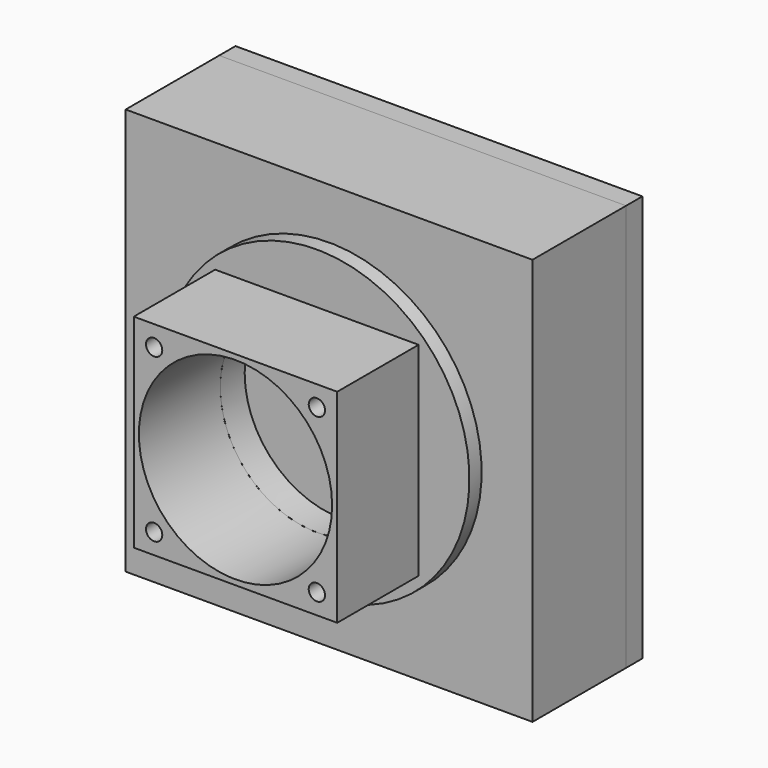
from build123d import *

# Parameters (mm, degrees)
F0_W      = 40
F0_H      = 40
F0_R      = 1.6
F0_R_2    = 19
F1_DEPTH  = 20
F2_R      = 30
F2_W      = 40
F2_H      = 40
F2_R_2    = 1.6
F2_R_3    = 19
F3_DEPTH  = 3
F4_W      = 80
F4_H      = 80
F4_R      = 30
F4_R_2    = 3
F4_R_3    = 19
F5_DEPTH  = 3
F6_W      = 80
F6_H      = 80
F6_W_2    = 76.0000017285
F6_H_2    = 76.0000017285
F7_DEPTH  = 20
F8_W      = 75.600002408
F8_H      = 75.600002408
F9_DEPTH  = 4
F8_W_2    = 80
F8_H_2    = 80
F8_W_3    = 76.0000017285
F8_H_3    = 76.0000017285
F10_DEPTH = 4


# Not quite as in the source:
# - a feature names something its author has since deleted; it is built from what else it names


with BuildPart() as f1:
    # F0 (on Front) → F1 (new body)
    with BuildSketch(Plane.XZ):
        Rectangle(F0_W, F0_H)
        with Locations((-16, -16)):
            Circle(F0_R, mode=Mode.SUBTRACT)
        with Locations((16, -16)):
            Circle(F0_R, mode=Mode.SUBTRACT)
        with Locations((-16, 16)):
            Circle(F0_R, mode=Mode.SUBTRACT)
        Circle(F0_R_2, mode=Mode.SUBTRACT)
        with Locations((16, 16)):
            Circle(F0_R, mode=Mode.SUBTRACT)
    extrude(amount=F1_DEPTH)


with BuildPart() as f3:
    # F2 (on face) → F3 (new body)
    with BuildSketch(Plane(origin=(0, 0, 0), x_dir=(-1, 0, 0), z_dir=(0, 1, 0))):
        Circle(F2_R)
        Rectangle(F2_W, F2_H, mode=Mode.SUBTRACT)
        Rectangle(F2_W, F2_H)
        with Locations((-16, -16)):
            Circle(F2_R_2, mode=Mode.SUBTRACT)
        with Locations((16, -16)):
            Circle(F2_R_2, mode=Mode.SUBTRACT)
        with Locations((-16, 16)):
            Circle(F2_R_2, mode=Mode.SUBTRACT)
        Circle(F2_R_3, mode=Mode.SUBTRACT)
        with Locations((16, 16)):
            Circle(F2_R_2, mode=Mode.SUBTRACT)
    extrude(amount=F3_DEPTH)

    # F4 (on face) → F5 (join)
    with BuildSketch(Plane(origin=(0, 3, 0), x_dir=(-1, 0, 0), z_dir=(0, 1, 0))):
        Rectangle(F4_W, F4_H)
        Circle(F4_R, mode=Mode.SUBTRACT)
        Circle(F4_R)
        with Locations((-16, -16)):
            Circle(F4_R_2, mode=Mode.SUBTRACT)
        with Locations((16, -16)):
            Circle(F4_R_2, mode=Mode.SUBTRACT)
        with Locations((-16, 16)):
            Circle(F4_R_2, mode=Mode.SUBTRACT)
        Circle(F4_R_3, mode=Mode.SUBTRACT)
        with Locations((16, 16)):
            Circle(F4_R_2, mode=Mode.SUBTRACT)
    extrude(amount=F5_DEPTH)

    # F6 (on face) → F7 (join)
    with BuildSketch(Plane(origin=(0, 6, 0), x_dir=(-1, 0, 0), z_dir=(0, 1, 0))):
        Rectangle(F6_W, F6_H)
        Rectangle(F6_W_2, F6_H_2, mode=Mode.SUBTRACT)
    extrude(amount=F7_DEPTH)


with BuildPart() as f9:
    # F8 (on face) → F9 (new body)
    with BuildSketch(Plane(origin=(0, 26, 0), x_dir=(-1, 0, 0), z_dir=(0, 1, 0))):
        Rectangle(F8_W, F8_H)
        with BuildLine():
            ThreePointArc((15.4, 11.1283421946), (18.0776104616, 5.8480766069), (19, 0))
            ThreePointArc((19, 0), (18.0776104616, -5.8480766069), (15.4, -11.1283421946))
            ThreePointArc((15.4, -11.1283421946), (15.0088486145, -11.6505134336), (14.6, -12.1589473229))
            ThreePointArc((14.6, -12.1589473229), (12.6392497246, -14.1862386276), (10.4, -15.9009433682))
            ThreePointArc((10.4, -15.9009433682), (10.0030672654, -16.153595429), (9.6, -16.3963410552))
            ThreePointArc((9.6, -16.3963410552), (7.5550130945, -17.4333524356), (5.4, -18.2164760588))
            ThreePointArc((5.4, -18.2164760588), (5.0011909438, -18.3299778817), (4.6, -18.4347497949))
            ThreePointArc((4.6, -18.4347497949), (2.5156890208, -18.8327191014), (0.4, -18.995789007))
            ThreePointArc((0.4, -18.995789007), (0, -19), (-0.4, -18.995789007))
            ThreePointArc((-0.4, -18.995789007), (-2.5156890208, -18.8327191014), (-4.6, -18.4347497949))
            ThreePointArc((-4.6, -18.4347497949), (-5.0011909438, -18.3299778817), (-5.4, -18.2164760588))
            ThreePointArc((-5.4, -18.2164760588), (-7.5550130945, -17.4333524356), (-9.6, -16.3963410552))
            ThreePointArc((-9.6, -16.3963410552), (-10.0030672654, -16.153595429), (-10.4, -15.9009433682))
            ThreePointArc((-10.4, -15.9009433682), (-12.6392497246, -14.1862386276), (-14.6, -12.1589473229))
            ThreePointArc((-14.6, -12.1589473229), (-15.0088486145, -11.6505134336), (-15.4, -11.1283421946))
            ThreePointArc((-15.4, -11.1283421946), (-19, 0), (-15.4, 11.1283421946))
            ThreePointArc((-15.4, 11.1283421946), (-15.0088486145, 11.6505134336), (-14.6, 12.1589473229))
            ThreePointArc((-14.6, 12.1589473229), (-12.6392497246, 14.1862386276), (-10.4, 15.9009433682))
            ThreePointArc((-10.4, 15.9009433682), (-10.0030672654, 16.153595429), (-9.6, 16.3963410552))
            ThreePointArc((-9.6, 16.3963410552), (-7.5550130945, 17.4333524356), (-5.4, 18.2164760588))
            ThreePointArc((-5.4, 18.2164760588), (-5.0011909438, 18.3299778817), (-4.6, 18.4347497949))
            ThreePointArc((-4.6, 18.4347497949), (-2.5156890208, 18.8327191014), (-0.4, 18.995789007))
            ThreePointArc((-0.4, 18.995789007), (0, 19), (0.4, 18.995789007))
            ThreePointArc((0.4, 18.995789007), (2.5156890208, 18.8327191014), (4.6, 18.4347497949))
            ThreePointArc((4.6, 18.4347497949), (5.0011909438, 18.3299778817), (5.4, 18.2164760588))
            ThreePointArc((5.4, 18.2164760588), (7.5550130945, 17.4333524356), (9.6, 16.3963410552))
            ThreePointArc((9.6, 16.3963410552), (10.0030672654, 16.153595429), (10.4, 15.9009433682))
            ThreePointArc((10.4, 15.9009433682), (12.6392497246, 14.1862386276), (14.6, 12.1589473229))
            ThreePointArc((14.6, 12.1589473229), (15.0088486145, 11.6505134336), (15.4, 11.1283421946))
        make_face(mode=Mode.SUBTRACT)
        with BuildLine():
            Line((-14.6, -12.1589473229), (-14.6, 12.1589473229))
            ThreePointArc((-14.6, 12.1589473229), (-15.0088486145, 11.6505134336), (-15.4, 11.1283421946))
            Line((-15.4, 11.1283421946), (-15.4, -11.1283421946))
            ThreePointArc((-15.4, -11.1283421946), (-15.0088486145, -11.6505134336), (-14.6, -12.1589473229))
        make_face()
        with BuildLine():
            Line((-9.6, -16.3963410552), (-9.6, 16.3963410552))
            ThreePointArc((-9.6, 16.3963410552), (-10.0030672654, 16.153595429), (-10.4, 15.9009433682))
            Line((-10.4, 15.9009433682), (-10.4, -15.9009433682))
            ThreePointArc((-10.4, -15.9009433682), (-10.0030672654, -16.153595429), (-9.6, -16.3963410552))
        make_face()
        with BuildLine():
            Line((-4.6, -18.4347497949), (-4.6, 18.4347497949))
            ThreePointArc((-4.6, 18.4347497949), (-5.0011909438, 18.3299778817), (-5.4, 18.2164760588))
            Line((-5.4, 18.2164760588), (-5.4, -18.2164760588))
            ThreePointArc((-5.4, -18.2164760588), (-5.0011909438, -18.3299778817), (-4.6, -18.4347497949))
        make_face()
        with BuildLine():
            Line((0.4, -18.995789007), (0.4, 18.995789007))
            ThreePointArc((0.4, 18.995789007), (0, 19), (-0.4, 18.995789007))
            Line((-0.4, 18.995789007), (-0.4, -18.995789007))
            ThreePointArc((-0.4, -18.995789007), (0, -19), (0.4, -18.995789007))
        make_face()
        with BuildLine():
            Line((5.4, -18.2164760588), (5.4, 18.2164760588))
            ThreePointArc((5.4, 18.2164760588), (5.0011909438, 18.3299778817), (4.6, 18.4347497949))
            Line((4.6, 18.4347497949), (4.6, -18.4347497949))
            ThreePointArc((4.6, -18.4347497949), (5.0011909438, -18.3299778817), (5.4, -18.2164760588))
        make_face()
        with BuildLine():
            Line((10.4, -15.9009433682), (10.4, 15.9009433682))
            ThreePointArc((10.4, 15.9009433682), (10.0030672654, 16.153595429), (9.6, 16.3963410552))
            Line((9.6, 16.3963410552), (9.6, -16.3963410552))
            ThreePointArc((9.6, -16.3963410552), (10.0030672654, -16.153595429), (10.4, -15.9009433682))
        make_face()
        with BuildLine():
            Line((15.4, -11.1283421946), (15.4, 11.1283421946))
            ThreePointArc((15.4, 11.1283421946), (15.0088486145, 11.6505134336), (14.6, 12.1589473229))
            Line((14.6, 12.1589473229), (14.6, -12.1589473229))
            ThreePointArc((14.6, -12.1589473229), (15.0088486145, -11.6505134336), (15.4, -11.1283421946))
        make_face()
    extrude(amount=-F9_DEPTH)

    # F8 (on face) → F10 (join)
    with BuildSketch(Plane(origin=(0, 26, 0), x_dir=(-1, 0, 0), z_dir=(0, 1, 0))):
        Rectangle(F8_W_2, F8_H_2)
        Rectangle(F8_W_3, F8_H_3, mode=Mode.SUBTRACT)
        Rectangle(F8_W_3, F8_H_3)
        Rectangle(F8_W, F8_H, mode=Mode.SUBTRACT)
        Rectangle(F8_W, F8_H)
        with BuildLine():
            ThreePointArc((15.4, 11.1283421946), (18.0776104616, 5.8480766069), (19, 0))
            ThreePointArc((19, 0), (18.0776104616, -5.8480766069), (15.4, -11.1283421946))
            ThreePointArc((15.4, -11.1283421946), (15.0088486145, -11.6505134336), (14.6, -12.1589473229))
            ThreePointArc((14.6, -12.1589473229), (12.6392497246, -14.1862386276), (10.4, -15.9009433682))
            ThreePointArc((10.4, -15.9009433682), (10.0030672654, -16.153595429), (9.6, -16.3963410552))
            ThreePointArc((9.6, -16.3963410552), (7.5550130945, -17.4333524356), (5.4, -18.2164760588))
            ThreePointArc((5.4, -18.2164760588), (5.0011909438, -18.3299778817), (4.6, -18.4347497949))
            ThreePointArc((4.6, -18.4347497949), (2.5156890208, -18.8327191014), (0.4, -18.995789007))
            ThreePointArc((0.4, -18.995789007), (0, -19), (-0.4, -18.995789007))
            ThreePointArc((-0.4, -18.995789007), (-2.5156890208, -18.8327191014), (-4.6, -18.4347497949))
            ThreePointArc((-4.6, -18.4347497949), (-5.0011909438, -18.3299778817), (-5.4, -18.2164760588))
            ThreePointArc((-5.4, -18.2164760588), (-7.5550130945, -17.4333524356), (-9.6, -16.3963410552))
            ThreePointArc((-9.6, -16.3963410552), (-10.0030672654, -16.153595429), (-10.4, -15.9009433682))
            ThreePointArc((-10.4, -15.9009433682), (-12.6392497246, -14.1862386276), (-14.6, -12.1589473229))
            ThreePointArc((-14.6, -12.1589473229), (-15.0088486145, -11.6505134336), (-15.4, -11.1283421946))
            ThreePointArc((-15.4, -11.1283421946), (-19, 0), (-15.4, 11.1283421946))
            ThreePointArc((-15.4, 11.1283421946), (-15.0088486145, 11.6505134336), (-14.6, 12.1589473229))
            ThreePointArc((-14.6, 12.1589473229), (-12.6392497246, 14.1862386276), (-10.4, 15.9009433682))
            ThreePointArc((-10.4, 15.9009433682), (-10.0030672654, 16.153595429), (-9.6, 16.3963410552))
            ThreePointArc((-9.6, 16.3963410552), (-7.5550130945, 17.4333524356), (-5.4, 18.2164760588))
            ThreePointArc((-5.4, 18.2164760588), (-5.0011909438, 18.3299778817), (-4.6, 18.4347497949))
            ThreePointArc((-4.6, 18.4347497949), (-2.5156890208, 18.8327191014), (-0.4, 18.995789007))
            ThreePointArc((-0.4, 18.995789007), (0, 19), (0.4, 18.995789007))
            ThreePointArc((0.4, 18.995789007), (2.5156890208, 18.8327191014), (4.6, 18.4347497949))
            ThreePointArc((4.6, 18.4347497949), (5.0011909438, 18.3299778817), (5.4, 18.2164760588))
            ThreePointArc((5.4, 18.2164760588), (7.5550130945, 17.4333524356), (9.6, 16.3963410552))
            ThreePointArc((9.6, 16.3963410552), (10.0030672654, 16.153595429), (10.4, 15.9009433682))
            ThreePointArc((10.4, 15.9009433682), (12.6392497246, 14.1862386276), (14.6, 12.1589473229))
            ThreePointArc((14.6, 12.1589473229), (15.0088486145, 11.6505134336), (15.4, 11.1283421946))
        make_face(mode=Mode.SUBTRACT)
        with BuildLine():
            Line((-9.6, -16.3963410552), (-9.6, 16.3963410552))
            ThreePointArc((-9.6, 16.3963410552), (-10.0030672654, 16.153595429), (-10.4, 15.9009433682))
            Line((-10.4, 15.9009433682), (-10.4, -15.9009433682))
            ThreePointArc((-10.4, -15.9009433682), (-10.0030672654, -16.153595429), (-9.6, -16.3963410552))
        make_face()
        with BuildLine():
            Line((-14.6, -12.1589473229), (-14.6, 12.1589473229))
            ThreePointArc((-14.6, 12.1589473229), (-15.0088486145, 11.6505134336), (-15.4, 11.1283421946))
            Line((-15.4, 11.1283421946), (-15.4, -11.1283421946))
            ThreePointArc((-15.4, -11.1283421946), (-15.0088486145, -11.6505134336), (-14.6, -12.1589473229))
        make_face()
        with BuildLine():
            Line((-4.6, -18.4347497949), (-4.6, 18.4347497949))
            ThreePointArc((-4.6, 18.4347497949), (-5.0011909438, 18.3299778817), (-5.4, 18.2164760588))
            Line((-5.4, 18.2164760588), (-5.4, -18.2164760588))
            ThreePointArc((-5.4, -18.2164760588), (-5.0011909438, -18.3299778817), (-4.6, -18.4347497949))
        make_face()
        with BuildLine():
            Line((0.4, -18.995789007), (0.4, 18.995789007))
            ThreePointArc((0.4, 18.995789007), (0, 19), (-0.4, 18.995789007))
            Line((-0.4, 18.995789007), (-0.4, -18.995789007))
            ThreePointArc((-0.4, -18.995789007), (0, -19), (0.4, -18.995789007))
        make_face()
        with BuildLine():
            Line((5.4, -18.2164760588), (5.4, 18.2164760588))
            ThreePointArc((5.4, 18.2164760588), (5.0011909438, 18.3299778817), (4.6, 18.4347497949))
            Line((4.6, 18.4347497949), (4.6, -18.4347497949))
            ThreePointArc((4.6, -18.4347497949), (5.0011909438, -18.3299778817), (5.4, -18.2164760588))
        make_face()
        with BuildLine():
            Line((10.4, -15.9009433682), (10.4, 15.9009433682))
            ThreePointArc((10.4, 15.9009433682), (10.0030672654, 16.153595429), (9.6, 16.3963410552))
            Line((9.6, 16.3963410552), (9.6, -16.3963410552))
            ThreePointArc((9.6, -16.3963410552), (10.0030672654, -16.153595429), (10.4, -15.9009433682))
        make_face()
        with BuildLine():
            Line((15.4, -11.1283421946), (15.4, 11.1283421946))
            ThreePointArc((15.4, 11.1283421946), (15.0088486145, 11.6505134336), (14.6, 12.1589473229))
            Line((14.6, 12.1589473229), (14.6, -12.1589473229))
            ThreePointArc((14.6, -12.1589473229), (15.0088486145, -11.6505134336), (15.4, -11.1283421946))
        make_face()
    extrude(amount=F10_DEPTH)


solid = Compound([f1.part, f3.part, f9.part])
